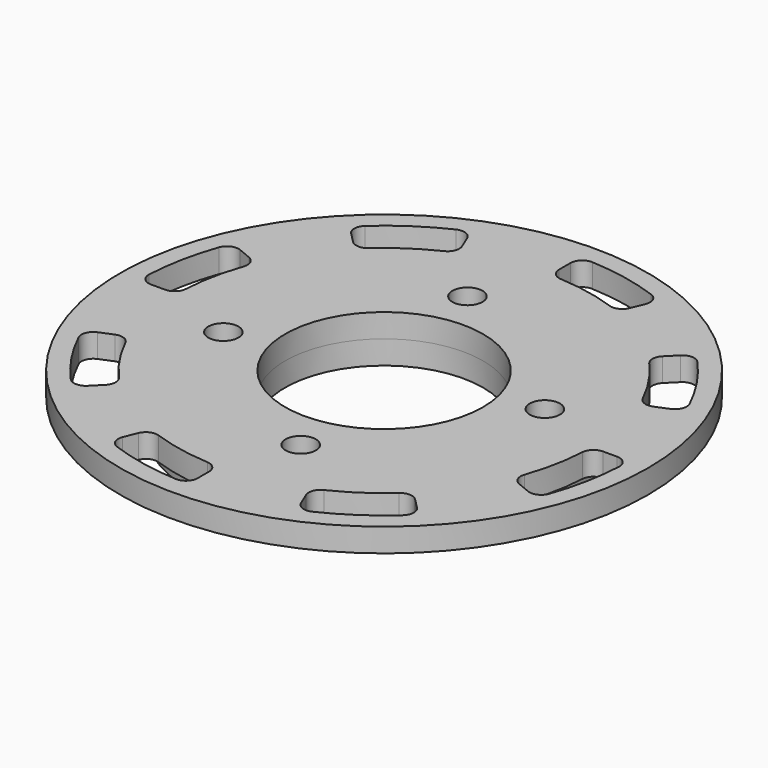
from build123d import *

# Parameters (mm, degrees)
F0_R     = 35.56
F0_R_2   = 25.4
F0_R_3   = 2.032
F0_R_4   = 13.335
F1_DEPTH = 3.175
F2_R     = 1.5875
F3_DEPTH = 3.175


# Not quite as in the source:
# - a feature names something its author has since deleted; it is built from what else it names


with BuildPart() as f1:
    # F0 (on Top) → F1 (new body)
    with BuildSketch(Plane.XY):
        Circle(F0_R)
        with BuildLine():
            ThreePointArc((-10.6921751003, -25.8131941384), (-5.4508235971, -27.4031407345), (0, -27.94))
            Line((0, -27.94), (0, -33.02))
            ThreePointArc((0, -33.02), (-6.441882433, -32.3855299589), (-12.6362069367, -30.5065021635))
            Line((-12.6362069367, -30.5065021635), (-10.6921751003, -25.8131941384))
        make_face(mode=Mode.SUBTRACT)
        with BuildLine():
            ThreePointArc((-25.8131941384, -10.6921751003), (-23.2312609677, -15.5226323106), (-19.7565634664, -19.7565634664))
            Line((-19.7565634664, -19.7565634664), (-23.3486659148, -23.3486659148))
            ThreePointArc((-23.3486659148, -23.3486659148), (-27.4551265982, -18.3449290943), (-30.5065021635, -12.6362069367))
            Line((-30.5065021635, -12.6362069367), (-25.8131941384, -10.6921751003))
        make_face(mode=Mode.SUBTRACT)
        Circle(F0_R_2, mode=Mode.SUBTRACT)
        with BuildLine():
            ThreePointArc((10.6921751003, -25.8131941384), (15.5226323106, -23.2312609677), (19.7565634664, -19.7565634664))
            Line((19.7565634664, -19.7565634664), (23.3486659148, -23.3486659148))
            ThreePointArc((23.3486659148, -23.3486659148), (18.3449290943, -27.4551265982), (12.6362069367, -30.5065021635))
            Line((12.6362069367, -30.5065021635), (10.6921751003, -25.8131941384))
        make_face(mode=Mode.SUBTRACT)
        with BuildLine():
            ThreePointArc((25.8131941384, -10.6921751003), (27.4031407345, -5.4508235971), (27.94, 0))
            Line((27.94, 0), (33.02, 0))
            ThreePointArc((33.02, 0), (32.3855299589, -6.441882433), (30.5065021635, -12.6362069367))
            Line((30.5065021635, -12.6362069367), (25.8131941384, -10.6921751003))
        make_face(mode=Mode.SUBTRACT)
        with BuildLine():
            ThreePointArc((-25.8131941384, 10.6921751003), (-27.4031407345, 5.4508235971), (-27.94, 0))
            Line((-27.94, 0), (-33.02, 0))
            ThreePointArc((-33.02, 0), (-32.3855299589, 6.441882433), (-30.5065021635, 12.6362069367))
            Line((-30.5065021635, 12.6362069367), (-25.8131941384, 10.6921751003))
        make_face(mode=Mode.SUBTRACT)
        with BuildLine():
            ThreePointArc((-10.6921751003, 25.8131941384), (-15.5226323106, 23.2312609677), (-19.7565634664, 19.7565634664))
            Line((-19.7565634664, 19.7565634664), (-23.3486659148, 23.3486659148))
            ThreePointArc((-23.3486659148, 23.3486659148), (-18.3449290943, 27.4551265982), (-12.6362069367, 30.5065021635))
            Line((-12.6362069367, 30.5065021635), (-10.6921751003, 25.8131941384))
        make_face(mode=Mode.SUBTRACT)
        with BuildLine():
            ThreePointArc((25.8131941384, 10.6921751003), (23.2312609677, 15.5226323106), (19.7565634664, 19.7565634664))
            Line((19.7565634664, 19.7565634664), (23.3486659148, 23.3486659148))
            ThreePointArc((23.3486659148, 23.3486659148), (27.4551265982, 18.3449290943), (30.5065021635, 12.6362069367))
            Line((30.5065021635, 12.6362069367), (25.8131941384, 10.6921751003))
        make_face(mode=Mode.SUBTRACT)
        with BuildLine():
            ThreePointArc((10.6921751003, 25.8131941384), (5.4508235971, 27.4031407345), (0, 27.94))
            Line((0, 27.94), (0, 33.02))
            ThreePointArc((0, 33.02), (6.441882433, 32.3855299589), (12.6362069367, 30.5065021635))
            Line((12.6362069367, 30.5065021635), (10.6921751003, 25.8131941384))
        make_face(mode=Mode.SUBTRACT)
        Circle(F0_R_2)
        with Locations((-18.6839595917, -3.7164706344)):
            Circle(F0_R_3, mode=Mode.SUBTRACT)
        Circle(F0_R_4, mode=Mode.SUBTRACT)
        with Locations((3.7164706344, -18.6839595917)):
            Circle(F0_R_3, mode=Mode.SUBTRACT)
        with Locations((-3.7164706344, 18.6839595917)):
            Circle(F0_R_3, mode=Mode.SUBTRACT)
        with Locations((18.6839595917, 3.7164706344)):
            Circle(F0_R_3, mode=Mode.SUBTRACT)
    extrude(amount=F1_DEPTH)

    # F2
    f2_edges = [f1.edges().sort_by_distance(p)[0] for p in [
        (-12.636207, 30.506502, 1.5875),
        (0, 33.02, 1.5875),
        (-19.756563, -19.756563, 1.5875),
        (-25.813194, 10.692175, 1.5875),
        (-23.348666, 23.348666, 1.5875),
        (-30.506502, 12.636207, 1.5875),
        (-25.813194, -10.692175, 1.5875),
        (0, 27.94, 1.5875),
        (10.692175, 25.813194, 1.5875),
        (-30.506502, -12.636207, 1.5875),
        (-33.02, 0, 1.5875),
        (-19.756563, 19.756563, 1.5875),
        (12.636207, 30.506502, 1.5875),
        (-23.348666, -23.348666, 1.5875),
        (-27.94, 0, 1.5875),
        (-10.692175, 25.813194, 1.5875),
        (23.348666, 23.348666, 1.5875),
        (27.94, 0, 1.5875),
        (19.756563, -19.756563, 1.5875),
        (-10.692175, -25.813194, 1.5875),
        (19.756563, 19.756563, 1.5875),
        (25.813194, -10.692175, 1.5875),
        (10.692175, -25.813194, 1.5875),
        (-12.636207, -30.506502, 1.5875),
        (25.813194, 10.692175, 1.5875),
        (30.506502, -12.636207, 1.5875),
        (12.636207, -30.506502, 1.5875),
        (30.506502, 12.636207, 1.5875),
        (23.348666, -23.348666, 1.5875),
        (33.02, 0, 1.5875),
        (0, -27.94, 1.5875),
        (0, -33.02, 1.5875),
    ]]
    fillet(f2_edges, radius=F2_R)


with BuildPart() as f3:
    # F0 (on Top) → F3 (new body)
    with BuildSketch(Plane.XY):
        Circle(F0_R_2)
        with Locations((-18.6839595917, -3.7164706344)):
            Circle(F0_R_3, mode=Mode.SUBTRACT)
        Circle(F0_R_4, mode=Mode.SUBTRACT)
        with Locations((3.7164706344, -18.6839595917)):
            Circle(F0_R_3, mode=Mode.SUBTRACT)
        with Locations((-3.7164706344, 18.6839595917)):
            Circle(F0_R_3, mode=Mode.SUBTRACT)
        with Locations((18.6839595917, 3.7164706344)):
            Circle(F0_R_3, mode=Mode.SUBTRACT)
    extrude(amount=-F3_DEPTH)


solid = Compound([f1.part, f3.part])
